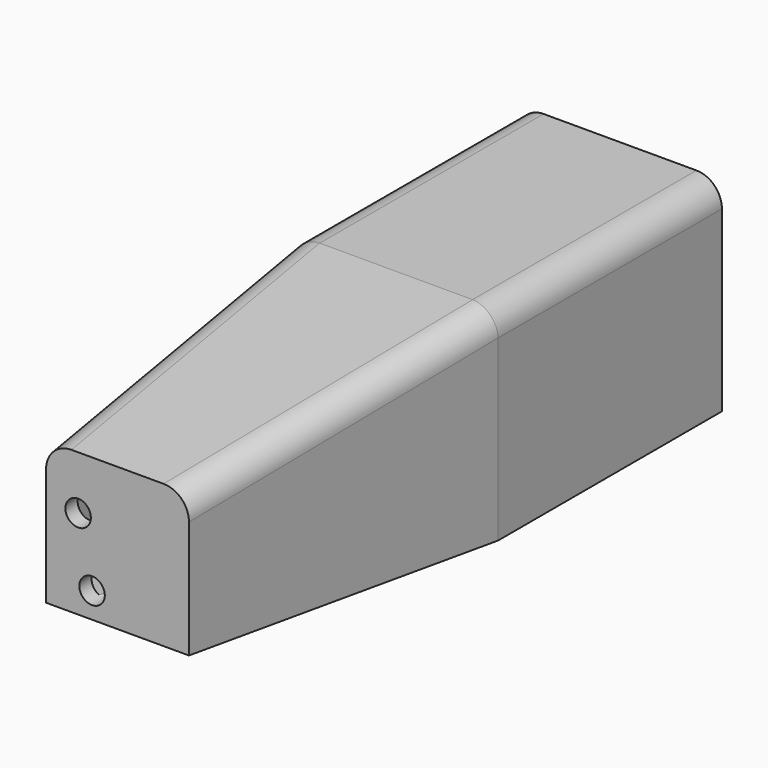
from build123d import *

# Parameters (mm, degrees)
F0_W          = 40
F0_H          = 40
F1_DEPTH      = 68.34402
F1_TAPER      = 5
F1_DEPTH_BACK = 54.92041
F2_T1_DEPTH   = 129.92041
F2_T3_DEPTH   = 143.2975946274
F2_T5_DEPTH   = 143.2975946274
F3_T          = 3
F5_D          = 5


# Not quite as in the source:
# - a fillet or chamfer that OpenCascade refuses, or shapes differently, is made with other operations: its cross-section is extruded or revolved along the edge and cut away or added
# - a shell that OpenCascade refuses in one call is made with other operations: the cavity is built on its own and cut out


with BuildPart() as f1:
    # F0 (on Front) → F1 (new body, two sides)
    with BuildSketch(Plane.XZ) as f1_sk:
        Rectangle(F0_W, F0_H)
    extrude(amount=F1_DEPTH, taper=F1_TAPER)
    extrude(f1_sk.sketch, amount=-F1_DEPTH_BACK)

    # F2: fillet of radius 5 on 4 edges, made by hand

    # F2_s2 → F2_t1 (cut)
    with BuildSketch(Plane.XZ.offset(-67.42041)):
        with BuildLine():
            ThreePointArc((20, 15), (18.5355339059, 18.5355339059), (15, 20))
            Line((15, 20), (20, 20))
            Line((20, 20), (20, 15))
        make_face()
        with BuildLine():
            ThreePointArc((-15, 20), (-18.5355339059, 18.5355339059), (-20, 15))
            Line((-20, 15), (-20, 20))
            Line((-20, 20), (-15, 20))
        make_face()
    extrude(amount=F2_T1_DEPTH, mode=Mode.SUBTRACT)

    # F2_s4 → F2_t3 (cut)
    with BuildSketch(Plane(origin=(5.6871501966, 65.0044242011, 5.6871501966), x_dir=(0.9961946981, -0.0871557427, 0), z_dir=(-0.0868265939, -0.9924325091, -0.0868265939))):
        with BuildLine():
            ThreePointArc((19.9238939618, 14.8109575307), (18.4728306397, 18.3330376627), (14.9618745793, 19.8108132759))
            Line((14.9618745793, 19.8108132759), (19.9238939618, 19.7731200764))
            Line((19.9238939618, 19.7731200764), (19.9238939618, 14.8109575307))
        make_face()
    extrude(amount=F2_T3_DEPTH, mode=Mode.SUBTRACT)

    # F2_s6 → F2_t5 (cut)
    with BuildSketch(Plane(origin=(-5.6871501966, 65.0044242011, 5.6871501966), x_dir=(0.9961946981, 0.0871557427, 0), z_dir=(0.0868265939, -0.9924325091, -0.0868265939))):
        with BuildLine():
            ThreePointArc((-14.9618745793, 19.8108132759), (-18.4728306397, 18.3330376627), (-19.9238939618, 14.8109575307))
            Line((-19.9238939618, 14.8109575307), (-19.9238939618, 19.7731200764))
            Line((-19.9238939618, 19.7731200764), (-14.9618745793, 19.8108132759))
        make_face()
    extrude(amount=F2_T5_DEPTH, mode=Mode.SUBTRACT)

    # F3: shell of thickness 3, made by hand


with BuildPart() as f3_core1:
    # F3_t2: copy of F1
    add(f1.part)

    # the walls: a layer under each face that stays
    f3_faces = [f3_core1.faces().sort_by_distance(p)[0] for p in [
        (20, 27.460205, -2.5),
        (17.0103365151, -34.17201, -2.1182047008),
        (18.5355339059, 27.415284207, 18.5355339059),
        (0, 27.460205, -20),
        (0, -34.17201, -17.0103365151),
        (0, -68.34402, -1.4566061483),
        (15.5420062021, -34.3060178162, 15.5420062021),
        (0, 27.460205, 20),
        (0, -34.17201, 17.0103365151),
        (-20, 27.460205, -2.5),
        (-18.5355339059, 27.415284207, 18.5355339059),
        (-17.0103365151, -34.17201, -2.1182047008),
        (-15.5420062021, -34.3060178161, 15.5420062021),
    ]]
    thicken(f3_faces, amount=-F3_T, mode=Mode.SUBTRACT)


with BuildPart() as f1_1:
    add(f1.part)

    # what is left inside the walls is the cavity
    f3_cavity = [f3_core1.part.solids().sort_by_distance(p)[0] for p in [
        (0, 36.657268, -16.97),
    ]]
    add(f3_cavity, mode=Mode.SUBTRACT)

    # F5 (through all)
    with Locations(Plane.XZ.offset(68.34402)):
        with Locations((-5, -9), (-7.7271993353, 3.5151276782)):
            Hole(F5_D / 2)


solid = f1_1.part
